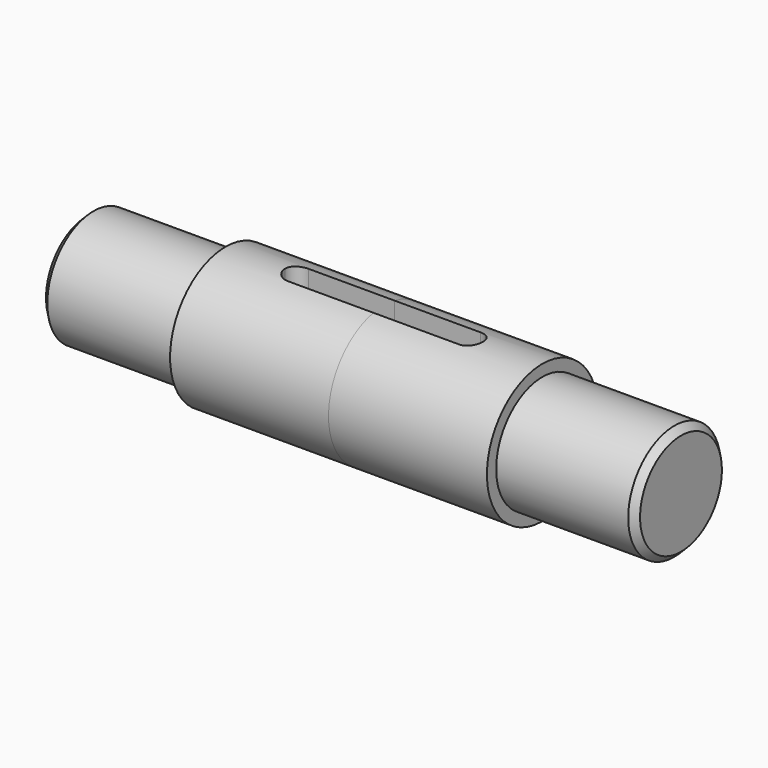
from build123d import *

# Parameters (mm, degrees)
F0_R     = 21
F1_DEPTH = 48
F2_R     = 17.5
F3_DEPTH = 42
F4_SIZE  = 2
F5_W     = 8
F5_H     = 12
F6_DEPTH = 30
F7_R     = 3.999


# Not quite as in the source:
# - a fillet or chamfer is up to 0.001 mm smaller than in the source, because OpenCascade refuses the exact size


with BuildPart() as f1:
    # F0 (on Right) → F1 (new body)
    with BuildSketch(Plane.YZ):
        Circle(F0_R)
    extrude(amount=F1_DEPTH)

    # F2 (on face) → F3 (join)
    with BuildSketch(Plane.YZ.offset(48)):
        Circle(F2_R)
    extrude(amount=F3_DEPTH)

    # F4
    f4_edges = [f1.edges().sort_by_distance(p)[0] for p in [
        (90, -17.5, 0),
    ]]
    chamfer(f4_edges, length=F4_SIZE)

    # F5 (on face) → F6 (cut)
    with BuildSketch(Plane(origin=(0, 0, 0), x_dir=(0, -1, 0), z_dir=(-1, 0, 0))):
        with Locations((0, 21)):
            Rectangle(F5_W, F5_H)
    extrude(amount=-F6_DEPTH, mode=Mode.SUBTRACT)

    # F7 (radius 4 in the source; OpenCascade refuses exactly that, so slightly less here)
    f7_edges = [f1.edges().sort_by_distance(p)[0] for p in [
        (30, 4, 17.807764),
        (30, -4, 17.807764),
    ]]
    fillet(f7_edges, radius=F7_R)

    # F8: F1 across face


with BuildPart() as f1_1:
    add(f1.part)
    add(f1.part.mirror(Plane(origin=(0, 0, -0.629577464), x_dir=(0, 1, 0), z_dir=(-1, 0, 0))))


solid = f1_1.part
